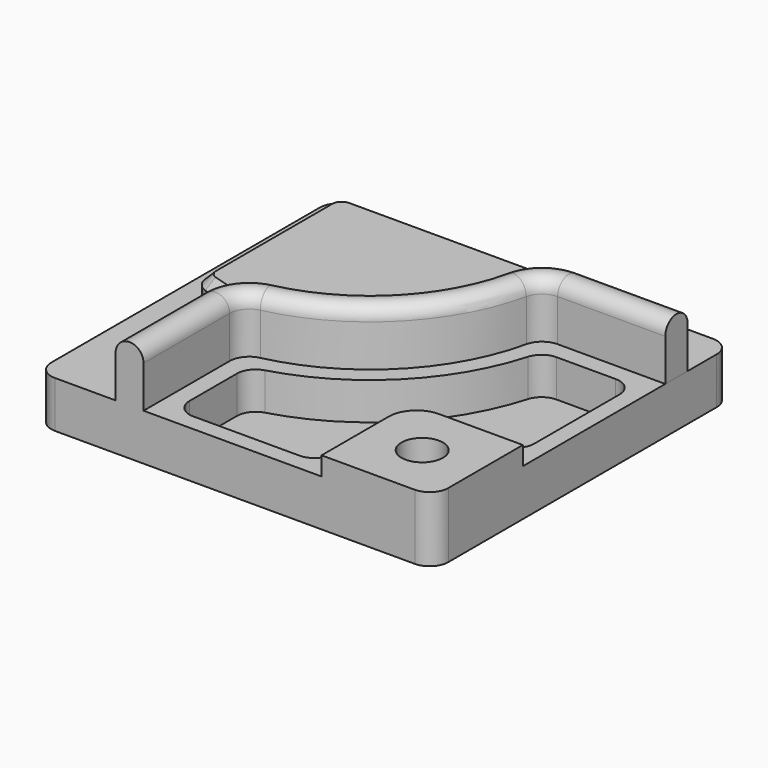
from build123d import *

# Parameters (mm, degrees)
F1_DEPTH       = 25
F2_DEPTH       = 10
F3_DEPTH       = 10
F4_DEPTH       = 20
F6_D           = 14.75
F6_CBORE_D     = 22.25
F6_CBORE_DEPTH = 14
F9_SIZE        = 5


with BuildPart() as f1:
    # F0 (on Top) → F1 (new body)
    with BuildSketch(Plane.XY):
        with BuildLine():
            Line((96.5, 100), (-96.5, 100))
            ThreePointArc((-96.5, 100), (-103.5710678119, 97.0710678119), (-106.5, 90))
            Line((-106.5, 90), (-106.5, -90))
            ThreePointArc((-106.5, -90), (-103.5710678119, -97.0710678119), (-96.5, -100))
            Line((-96.5, -100), (-63.5, -100))
            Line((-63.5, -100), (-63.5, -42.2497216032))
            ThreePointArc((-63.5, -42.2497216032), (-58.0047374401, -26.6111405489), (-43.9347826087, -17.8476082112))
            ThreePointArc((-43.9347826087, -17.8476082112), (0.1396103068, 6.3603896932), (24.3476082112, 50.4347826087))
            ThreePointArc((24.3476082112, 50.4347826087), (33.1111405489, 64.5047374401), (48.7497216032, 70))
            Line((48.7497216032, 70), (106.5, 70))
            Line((106.5, 70), (106.5, 90))
            ThreePointArc((106.5, 90), (103.5710678119, 97.0710678119), (96.5, 100))
        make_face()
        with BuildLine():
            ThreePointArc((17.5, 70), (-16.8995859294, 3.7474422497), (-90.8802816901, -6.2320154172))
            ThreePointArc((-90.8802816901, -6.2320154172), (-95.6793281173, -2.5737930287), (-97.5, 3.1793445108))
            Line((-97.5, 3.1793445108), (-97.5, 81))
            ThreePointArc((-97.5, 81), (-94.5710678119, 88.0710678119), (-87.5, 91))
            Line((-87.5, 91), (7.5, 91))
            ThreePointArc((7.5, 91), (14.5710678119, 88.0710678119), (17.5, 81))
            Line((17.5, 81), (17.5, 70))
        make_face(mode=Mode.SUBTRACT)
        with BuildLine():
            Line((106.5, 55), (106.5, 70))
            Line((106.5, 70), (48.7497216032, 70))
            ThreePointArc((48.7497216032, 70), (33.1111405489, 64.5047374401), (24.3476082112, 50.4347826087))
            ThreePointArc((24.3476082112, 50.4347826087), (0.1396103068, 6.3603896932), (-43.9347826087, -17.8476082112))
            ThreePointArc((-43.9347826087, -17.8476082112), (-58.0047374401, -26.6111405489), (-63.5, -42.2497216032))
            Line((-63.5, -42.2497216032), (-63.5, -100))
            Line((-63.5, -100), (-48.5, -100))
            Line((-48.5, -100), (-48.5, -42.2497216032))
            ThreePointArc((-48.5, -42.2497216032), (-46.3018949761, -35.9942891815), (-40.6739130435, -32.4888762464))
            ThreePointArc((-40.6739130435, -32.4888762464), (10.7462120246, -4.2462120246), (38.9888762464, 47.1739130435))
            ThreePointArc((38.9888762464, 47.1739130435), (42.4942891815, 52.8018949761), (48.7497216032, 55))
            Line((48.7497216032, 55), (106.5, 55))
        make_face()
        with BuildLine():
            Line((106.5, -40), (106.5, 55))
            Line((106.5, 55), (48.7497216032, 55))
            ThreePointArc((48.7497216032, 55), (42.4942891815, 52.8018949761), (38.9888762464, 47.1739130435))
            ThreePointArc((38.9888762464, 47.1739130435), (10.7462120246, -4.2462120246), (-40.6739130435, -32.4888762464))
            ThreePointArc((-40.6739130435, -32.4888762464), (-46.3018949761, -35.9942891815), (-48.5, -42.2497216032))
            Line((-48.5, -42.2497216032), (-48.5, -100))
            Line((-48.5, -100), (46.5, -100))
            Line((46.5, -100), (46.5, -55))
            ThreePointArc((46.5, -55), (50.8933982822, -44.3933982822), (61.5, -40))
            Line((61.5, -40), (106.5, -40))
        make_face()
        with BuildLine():
            Line((87.5, -31), (61.5, -31))
            ThreePointArc((61.5, -31), (44.5294372515, -38.0294372515), (37.5, -55))
            Line((37.5, -55), (37.5, -81))
            ThreePointArc((37.5, -81), (34.5710678119, -88.0710678119), (27.5, -91))
            Line((27.5, -91), (-29.5, -91))
            ThreePointArc((-29.5, -91), (-36.5710678119, -88.0710678119), (-39.5, -81))
            Line((-39.5, -81), (-39.5, -49.2476414861))
            ThreePointArc((-39.5, -49.2476414861), (-37.481834214, -43.2234965193), (-32.2419354839, -39.630896205))
            ThreePointArc((-32.2419354839, -39.630896205), (17.1101730553, -10.6101730553), (46.130896205, 38.7419354839))
            ThreePointArc((46.130896205, 38.7419354839), (49.7234965193, 43.981834214), (55.7476414861, 46))
            Line((55.7476414861, 46), (87.5, 46))
            ThreePointArc((87.5, 46), (94.5710678119, 43.0710678119), (97.5, 36))
            Line((97.5, 36), (97.5, -21))
            ThreePointArc((97.5, -21), (94.5710678119, -28.0710678119), (87.5, -31))
        make_face(mode=Mode.SUBTRACT)
        with BuildLine():
            Line((106.5, -90), (106.5, -40))
            Line((106.5, -40), (61.5, -40))
            ThreePointArc((61.5, -40), (50.8933982822, -44.3933982822), (46.5, -55))
            Line((46.5, -55), (46.5, -100))
            Line((46.5, -100), (96.5, -100))
            ThreePointArc((96.5, -100), (103.5710678119, -97.0710678119), (106.5, -90))
        make_face()
        with BuildLine():
            ThreePointArc((-97.5, 3.1793445108), (-95.6793281173, -2.5737930287), (-90.8802816901, -6.2320154172))
            ThreePointArc((-90.8802816901, -6.2320154172), (-16.8995859294, 3.7474422497), (17.5, 70))
            Line((17.5, 70), (17.5, 81))
            ThreePointArc((17.5, 81), (14.5710678119, 88.0710678119), (7.5, 91))
            Line((7.5, 91), (-87.5, 91))
            ThreePointArc((-87.5, 91), (-94.5710678119, 88.0710678119), (-97.5, 81))
            Line((-97.5, 81), (-97.5, 3.1793445108))
        make_face()
        with BuildLine():
            ThreePointArc((37.5, -55), (44.5294372515, -38.0294372515), (61.5, -31))
            Line((61.5, -31), (87.5, -31))
            ThreePointArc((87.5, -31), (94.5710678119, -28.0710678119), (97.5, -21))
            Line((97.5, -21), (97.5, 36))
            ThreePointArc((97.5, 36), (94.5710678119, 43.0710678119), (87.5, 46))
            Line((87.5, 46), (55.7476414861, 46))
            ThreePointArc((55.7476414861, 46), (49.7234965193, 43.981834214), (46.130896205, 38.7419354839))
            ThreePointArc((46.130896205, 38.7419354839), (17.1101730553, -10.6101730553), (-32.2419354839, -39.630896205))
            ThreePointArc((-32.2419354839, -39.630896205), (-37.481834214, -43.2234965193), (-39.5, -49.2476414861))
            Line((-39.5, -49.2476414861), (-39.5, -81))
            ThreePointArc((-39.5, -81), (-36.5710678119, -88.0710678119), (-29.5, -91))
            Line((-29.5, -91), (27.5, -91))
            ThreePointArc((27.5, -91), (34.5710678119, -88.0710678119), (37.5, -81))
            Line((37.5, -81), (37.5, -55))
        make_face()
    extrude(amount=-F1_DEPTH)

    # F0 (on Top) → F2 (join)
    with BuildSketch(Plane.XY):
        with BuildLine():
            Line((106.5, -90), (106.5, -40))
            Line((106.5, -40), (61.5, -40))
            ThreePointArc((61.5, -40), (50.8933982822, -44.3933982822), (46.5, -55))
            Line((46.5, -55), (46.5, -100))
            Line((46.5, -100), (96.5, -100))
            ThreePointArc((96.5, -100), (103.5710678119, -97.0710678119), (106.5, -90))
        make_face()
    extrude(amount=F2_DEPTH)

    # F0 (on Top) → F3 (join)
    with BuildSketch(Plane.XY):
        with BuildLine():
            ThreePointArc((-97.5, 3.1793445108), (-95.6793281173, -2.5737930287), (-90.8802816901, -6.2320154172))
            ThreePointArc((-90.8802816901, -6.2320154172), (-16.8995859294, 3.7474422497), (17.5, 70))
            Line((17.5, 70), (17.5, 81))
            ThreePointArc((17.5, 81), (14.5710678119, 88.0710678119), (7.5, 91))
            Line((7.5, 91), (-87.5, 91))
            ThreePointArc((-87.5, 91), (-94.5710678119, 88.0710678119), (-97.5, 81))
            Line((-97.5, 81), (-97.5, 3.1793445108))
        make_face()
    extrude(amount=F3_DEPTH)

    # F0 (on Top) → F4 (cut)
    with BuildSketch(Plane.XY):
        with BuildLine():
            ThreePointArc((37.5, -55), (44.5294372515, -38.0294372515), (61.5, -31))
            Line((61.5, -31), (87.5, -31))
            ThreePointArc((87.5, -31), (94.5710678119, -28.0710678119), (97.5, -21))
            Line((97.5, -21), (97.5, 36))
            ThreePointArc((97.5, 36), (94.5710678119, 43.0710678119), (87.5, 46))
            Line((87.5, 46), (55.7476414861, 46))
            ThreePointArc((55.7476414861, 46), (49.7234965193, 43.981834214), (46.130896205, 38.7419354839))
            ThreePointArc((46.130896205, 38.7419354839), (17.1101730553, -10.6101730553), (-32.2419354839, -39.630896205))
            ThreePointArc((-32.2419354839, -39.630896205), (-37.481834214, -43.2234965193), (-39.5, -49.2476414861))
            Line((-39.5, -49.2476414861), (-39.5, -81))
            ThreePointArc((-39.5, -81), (-36.5710678119, -88.0710678119), (-29.5, -91))
            Line((-29.5, -91), (27.5, -91))
            ThreePointArc((27.5, -91), (34.5710678119, -88.0710678119), (37.5, -81))
            Line((37.5, -81), (37.5, -55))
        make_face()
    extrude(amount=-F4_DEPTH, mode=Mode.SUBTRACT)

    # F6 (through all)
    with Locations(Plane.XY.offset(10)):
        with Locations((76.5, -70)):
            CounterBoreHole(F6_D / 2, F6_CBORE_D / 2, F6_CBORE_DEPTH)

    # F8: sweep along a path in F0
    with BuildLine(Plane.XY) as f8_path:
        Line((-48.5, -100), (-48.5, -42.2497216032))
        ThreePointArc((-48.5, -42.2497216032), (-46.3018949761, -35.9942891815), (-40.6739130435, -32.4888762464))
        ThreePointArc((-40.6739130435, -32.4888762464), (10.7462120246, -4.2462120246), (38.9888762464, 47.1739130435))
        ThreePointArc((38.9888762464, 47.1739130435), (42.4942891815, 52.8018949761), (48.7497216032, 55))
        Line((48.7497216032, 55), (106.5, 55))
    # F7 (on face) → F8 (sweep)
    with BuildSketch(Plane.XZ.offset(100)):
        with BuildLine():
            Line((-64, 0), (-49, 0))
            Line((-49, 0), (-49, 22.5))
            ThreePointArc((-49, 22.5), (-56.5, 30), (-64, 22.5))
            Line((-64, 22.5), (-64, 0))
        make_face()
    sweep(path=f8_path.line)

    # F9
    f9_edges = [f1.edges().sort_by_distance(p)[0] for p in [
        (-97.5, 42.089672, 10),
    ]]
    chamfer(f9_edges, length=F9_SIZE)


solid = f1.part
